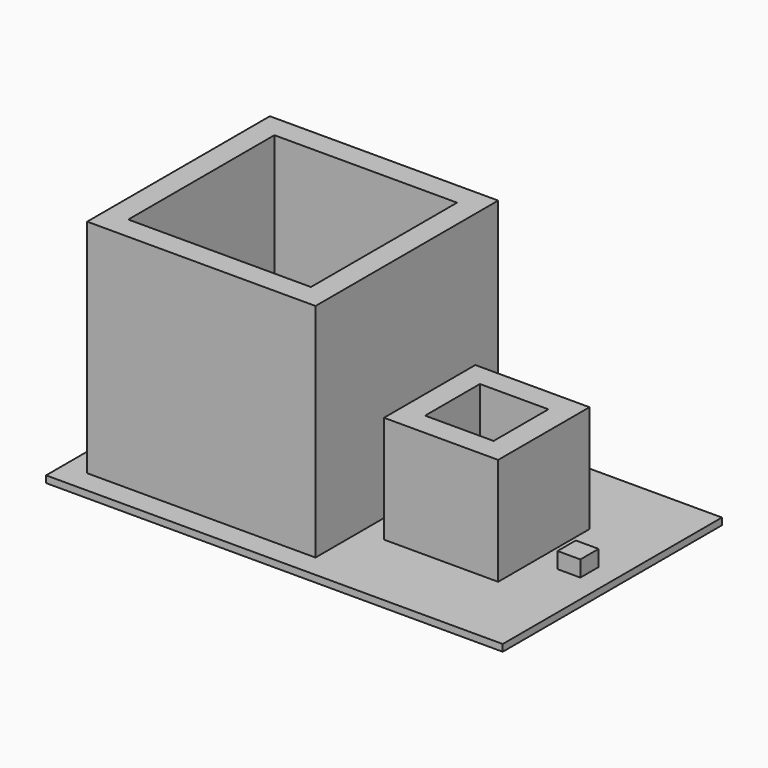
from build123d import *

# Parameters (mm, degrees)
F0_W         = 10
F0_H         = 10
F1_DEPTH     = 10
F0_W_2       = 5
F0_H_2       = 5
F2_DEPTH     = 5
F0_W_3       = 1
F0_H_3       = 1
F3_DEPTH     = 1
F0_W_4       = 20
F0_H_4       = 12
F4_DEPTH     = 0.3
F5_T         = 1
F5_T3_DEPTH  = 3
F5_T5_DEPTH  = 12
F5_T7_DEPTH  = 12
F5_T9_DEPTH  = 7
F5_T11_DEPTH = 7
F5_T13_DEPTH = 3


# Not quite as in the source:
# - a shell that OpenCascade refuses in one call is made with other operations: the cavity is built on its own and cut out


with BuildPart() as f1:
    # F0 (on Top) → F1 (new body)
    with BuildSketch(Plane.XY):
        Rectangle(F0_W, F0_H)
    extrude(amount=F1_DEPTH)



with BuildPart() as f2:
    # F0 (on Top) → F2 (new body)
    with BuildSketch(Plane.XY):
        with Locations((8.5, 0)):
            Rectangle(F0_W_2, F0_H_2)
    extrude(amount=F2_DEPTH)


with BuildPart() as f3:
    # F0 (on Top) → F3 (new body)
    with BuildSketch(Plane.XY):
        with Locations((12.5, 0)):
            Rectangle(F0_W_3, F0_H_3)
    extrude(amount=F3_DEPTH)


with BuildPart() as f1_1:
    add(f1.part)

    add(f2.part)  # F4 merges F2

    add(f3.part)  # F4 merges F3
    # F0 (on Top) → F4 (join)
    with BuildSketch(Plane.XY):
        with Locations((4, 0)):
            Rectangle(F0_W_4, F0_H_4)
        Rectangle(F0_W, F0_H, mode=Mode.SUBTRACT)
        with Locations((8.5, 0)):
            Rectangle(F0_W_2, F0_H_2, mode=Mode.SUBTRACT)
        with Locations((12.5, 0)):
            Rectangle(F0_W_3, F0_H_3, mode=Mode.SUBTRACT)
    extrude(amount=F4_DEPTH)

    # F5: shell of thickness 1, made by hand


with BuildPart() as f5_core1:
    # F5_t2: copy of F1
    add(f1_1.part)

    # the walls: a layer under each face that stays
    f5_faces = [f5_core1.faces().sort_by_distance(p)[0] for p in [
        (13, 0, 0.65),
        (10.6666666667, -4, 0.3),
        (12.5, 0.5, 0.65),
        (12.5, -0.5, 0.65),
        (4, 6, 0.15),
        (-6, 0, 0.15),
        (4, -6, 0.15),
        (14, 0, 0.15),
        (0, 5, 5.15),
        (5, 0, 5.15),
        (0, -5, 5.15),
        (-5, 0, 5.15),
        (8.5, 2.5, 2.65),
        (11, 0, 2.65),
        (8.5, -2.5, 2.65),
        (6, 0, 2.65),
        (12, 0, 0.65),
        (4, 0, 0),
    ]]
    thicken(f5_faces, amount=-F5_T, mode=Mode.SUBTRACT)

    # F5_s4 → F5_t3 (cut)
    with BuildSketch(Plane.XZ.offset(-1.5)):
        Polygon((13.01, 0.31), (12, 0.3), (12, -0.7), (13, -0.7), align=None)
        Polygon((11.99, 0.31), (12, -0.7), (13, -0.7), (13, 0.3), align=None)
    extrude(amount=F5_T3_DEPTH, mode=Mode.SUBTRACT)

    # F5_s6 → F5_t5 (cut)
    with BuildSketch(Plane.YZ.offset(-6)):
        Polygon((5.01, 0.31), (5, -0.7), (4, -0.7), (4, 0.3), align=None)
        Polygon((-5.01, 0.31), (-5, -0.7), (-4, -0.7), (-4, 0.3), align=None)
    extrude(amount=F5_T5_DEPTH, mode=Mode.SUBTRACT)

    # F5_s8 → F5_t7 (cut)
    with BuildSketch(Plane.XZ.offset(-6)):
        Polygon((5.01, 0.31), (5, -0.7), (4, -0.7), (4, 0.3), align=None)
        Polygon((-5.01, 0.31), (-5, -0.7), (-4, -0.7), (-4, 0.3), align=None)
    extrude(amount=F5_T7_DEPTH, mode=Mode.SUBTRACT)

    # F5_s10 → F5_t9 (cut)
    with BuildSketch(Plane.YZ.offset(5)):
        Polygon((2.51, 0.31), (2.5, -0.7), (1.5, -0.7), (1.5, 0.3), align=None)
        Polygon((-2.51, 0.31), (-2.5, -0.7), (-1.5, -0.7), (-1.5, 0.3), align=None)
    extrude(amount=F5_T9_DEPTH, mode=Mode.SUBTRACT)

    # F5_s12 → F5_t11 (cut)
    with BuildSketch(Plane.XZ.offset(-3.5)):
        Polygon((11.01, 0.31), (11, -0.7), (10, -0.7), (10, 0.3), align=None)
        Polygon((5.99, 0.31), (6, -0.7), (7, -0.7), (7, 0.3), align=None)
    extrude(amount=F5_T11_DEPTH, mode=Mode.SUBTRACT)

    # F5_s14 → F5_t13 (cut)
    with BuildSketch(Plane.YZ.offset(11)):
        Polygon((0.51, 0.31), (0.5, -0.7), (-0.5, -0.7), (-0.5, 0.3), align=None)
        Polygon((-0.51, 0.31), (-0.5, -0.7), (0.5, -0.7), (0.5, 0.3), align=None)
    extrude(amount=F5_T13_DEPTH, mode=Mode.SUBTRACT)


with BuildPart() as f1_2:
    add(f1_1.part)

    # what is left inside the walls is the cavity
    f5_cavity = [f5_core1.part.solids().sort_by_distance(p)[0] for p in [
        (3.99, 0, 7),
        (8.5, 1.49, 3.666667),
    ]]
    add(f5_cavity, mode=Mode.SUBTRACT)


solid = f1_2.part
